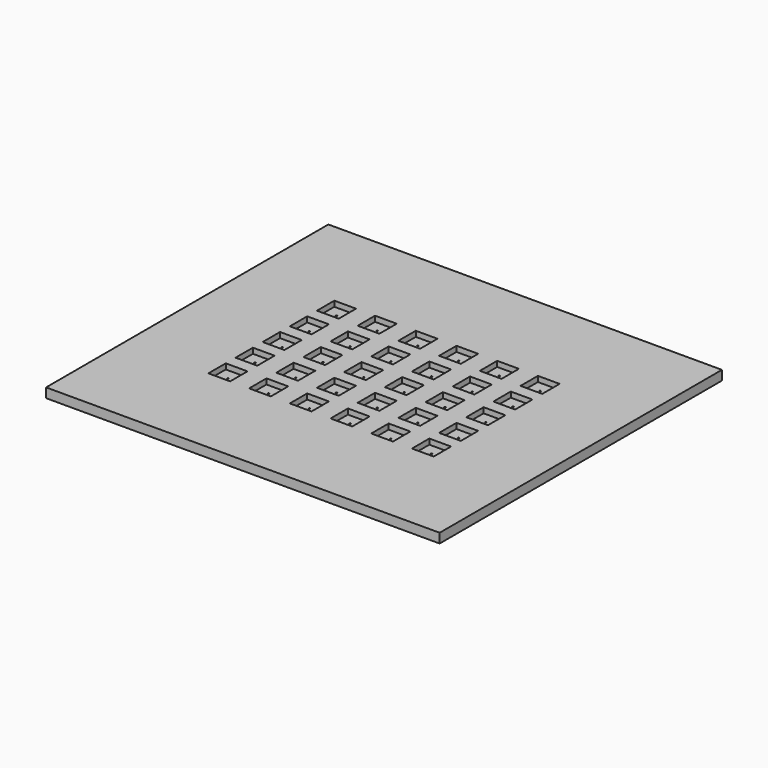
from build123d import *

# Parameters (mm, degrees)
F0_W     = 29
F0_H     = 26
F1_DEPTH = 0.7
F3_W     = 1.6
F3_H     = 1.6
F4_DEPTH = 0.4
F6_D     = 0.1
F8_D     = 0.1
F10_D    = 0.1
F12_D    = 0.1
F14_D    = 0.1
F16_D    = 0.1
F18_D    = 0.1
F20_D    = 0.1
F22_D    = 0.1
F24_D    = 0.1
F26_D    = 0.1
F28_D    = 0.1
F30_D    = 0.1
F32_D    = 0.1
F34_D    = 0.1
F36_D    = 0.1
F38_D    = 0.1
F40_D    = 0.1
F42_D    = 0.1
F44_D    = 0.1
F46_D    = 0.1
F48_D    = 0.1
F50_D    = 0.1
F52_D    = 0.1
F54_D    = 0.1
F56_D    = 0.1
F58_D    = 0.1
F60_D    = 0.1
F62_D    = 0.1
F64_D    = 0.1


# Not quite as in the source:
# - a feature names something its author has since deleted; it is built from what else it names


with BuildPart() as f1:
    # F0 (on Top) → F1 (new body)
    with BuildSketch(Plane.XY):
        Rectangle(F0_W, F0_H)
    extrude(amount=-F1_DEPTH)

    # F3 (on face) → F4 (cut)
    with BuildSketch(Plane.XY):
        with Locations((-7.5, 5)):
            Rectangle(F3_W, F3_H)
        with Locations((-4.5, 5)):
            Rectangle(F3_W, F3_H)
        with Locations((-1.5, 5)):
            Rectangle(F3_W, F3_H)
        with Locations((1.5, 5)):
            Rectangle(F3_W, F3_H)
        with Locations((4.5, 5)):
            Rectangle(F3_W, F3_H)
        with Locations((7.5, 5)):
            Rectangle(F3_W, F3_H)
        with Locations((-7.5, 2.5)):
            Rectangle(F3_W, F3_H)
        with Locations((-4.5, 2.5)):
            Rectangle(F3_W, F3_H)
        with Locations((-1.5, 2.5)):
            Rectangle(F3_W, F3_H)
        with Locations((1.5, 2.5)):
            Rectangle(F3_W, F3_H)
        with Locations((4.5, 2.5)):
            Rectangle(F3_W, F3_H)
        with Locations((7.5, 2.5)):
            Rectangle(F3_W, F3_H)
        with Locations((-7.5, 0)):
            Rectangle(F3_W, F3_H)
        with Locations((-4.5, 0)):
            Rectangle(F3_W, F3_H)
        with Locations((-1.5, 0)):
            Rectangle(F3_W, F3_H)
        with Locations((1.5, 0)):
            Rectangle(F3_W, F3_H)
        with Locations((4.5, 0)):
            Rectangle(F3_W, F3_H)
        with Locations((7.5, 0)):
            Rectangle(F3_W, F3_H)
        with Locations((-7.5, -2.5)):
            Rectangle(F3_W, F3_H)
        with Locations((-4.5, -2.5)):
            Rectangle(F3_W, F3_H)
        with Locations((-1.5, -2.5)):
            Rectangle(F3_W, F3_H)
        with Locations((1.5, -2.5)):
            Rectangle(F3_W, F3_H)
        with Locations((4.5, -2.5)):
            Rectangle(F3_W, F3_H)
        with Locations((7.5, -2.5)):
            Rectangle(F3_W, F3_H)
        with Locations((-7.5, -5)):
            Rectangle(F3_W, F3_H)
        with Locations((-4.5, -5)):
            Rectangle(F3_W, F3_H)
        with Locations((-1.5, -5)):
            Rectangle(F3_W, F3_H)
        with Locations((1.5, -5)):
            Rectangle(F3_W, F3_H)
        with Locations((4.5, -5)):
            Rectangle(F3_W, F3_H)
        with Locations((7.5, -5)):
            Rectangle(F3_W, F3_H)
    extrude(amount=-F4_DEPTH, mode=Mode.SUBTRACT)

    # F6 (through all)
    with Locations(Plane.XY.offset(-0.4)):
        with Locations((-7.5, 5)):
            Hole(F6_D / 2)

    # F8 (through all)
    with Locations(Plane.XY.offset(-0.4)):
        with Locations((-4.5, 5)):
            Hole(F8_D / 2)

    # F10 (through all)
    with Locations(Plane.XY.offset(-0.4)):
        with Locations((-1.5, 5)):
            Hole(F10_D / 2)

    # F12 (through all)
    with Locations(Plane.XY.offset(-0.4)):
        with Locations((1.5, 5)):
            Hole(F12_D / 2)

    # F14 (through all)
    with Locations(Plane.XY.offset(-0.4)):
        with Locations((4.5, 5)):
            Hole(F14_D / 2)

    # F16 (through all)
    with Locations(Plane.XY.offset(-0.4)):
        with Locations((7.5, 5)):
            Hole(F16_D / 2)

    # F18 (through all)
    with Locations(Plane.XY.offset(-0.4)):
        with Locations((7.5, 2.5)):
            Hole(F18_D / 2)

    # F20 (through all)
    with Locations(Plane.XY.offset(-0.4)):
        with Locations((4.5, 2.5)):
            Hole(F20_D / 2)

    # F22 (through all)
    with Locations(Plane.XY.offset(-0.4)):
        with Locations((1.5, 2.5)):
            Hole(F22_D / 2)

    # F24 (through all)
    with Locations(Plane.XY.offset(-0.4)):
        with Locations((-1.5, 2.5)):
            Hole(F24_D / 2)

    # F26 (through all)
    with Locations(Plane.XY.offset(-0.4)):
        with Locations((-4.5, 2.5)):
            Hole(F26_D / 2)

    # F28 (through all)
    with Locations(Plane.XY.offset(-0.4)):
        with Locations((-7.5, 2.5)):
            Hole(F28_D / 2)

    # F30 (through all)
    with Locations(Plane.XY.offset(-0.4)):
        with Locations((-7.5, 0)):
            Hole(F30_D / 2)

    # F32 (through all)
    with Locations(Plane.XY.offset(-0.4)):
        with Locations((-4.5, 0)):
            Hole(F32_D / 2)

    # F34 (through all)
    with Locations(Plane.XY.offset(-0.4)):
        with Locations((-1.5, 0)):
            Hole(F34_D / 2)

    # F36 (through all)
    with Locations(Plane.XY.offset(-0.4)):
        with Locations((1.5, 0)):
            Hole(F36_D / 2)

    # F38 (through all)
    with Locations(Plane.XY.offset(-0.4)):
        with Locations((4.5, 0)):
            Hole(F38_D / 2)

    # F40 (through all)
    with Locations(Plane.XY.offset(-0.4)):
        with Locations((7.5, 0)):
            Hole(F40_D / 2)

    # F42 (through all)
    with Locations(Plane.XY.offset(-0.4)):
        with Locations((-7.5, -2.5)):
            Hole(F42_D / 2)

    # F44 (through all)
    with Locations(Plane.XY.offset(-0.4)):
        with Locations((-4.5, -2.5)):
            Hole(F44_D / 2)

    # F46 (through all)
    with Locations(Plane.XY.offset(-0.4)):
        with Locations((-1.5, -2.5)):
            Hole(F46_D / 2)

    # F48 (through all)
    with Locations(Plane.XY.offset(-0.4)):
        with Locations((1.5, -2.5)):
            Hole(F48_D / 2)

    # F50 (through all)
    with Locations(Plane.XY.offset(-0.4)):
        with Locations((4.5, -2.5)):
            Hole(F50_D / 2)

    # F52 (through all)
    with Locations(Plane.XY.offset(-0.4)):
        with Locations((7.5, -2.5)):
            Hole(F52_D / 2)

    # F54 (through all)
    with Locations(Plane.XY.offset(-0.4)):
        with Locations((7.5, -5)):
            Hole(F54_D / 2)

    # F56 (through all)
    with Locations(Plane.XY.offset(-0.4)):
        with Locations((4.5, -5)):
            Hole(F56_D / 2)

    # F58 (through all)
    with Locations(Plane.XY.offset(-0.4)):
        with Locations((1.5, -5)):
            Hole(F58_D / 2)

    # F60 (through all)
    with Locations(Plane.XY.offset(-0.4)):
        with Locations((-1.5, -5)):
            Hole(F60_D / 2)

    # F62 (through all)
    with Locations(Plane.XY.offset(-0.4)):
        with Locations((-4.5, -5)):
            Hole(F62_D / 2)

    # F64 (through all)
    with Locations(Plane.XY.offset(-0.4)):
        with Locations((-7.5, -5)):
            Hole(F64_D / 2)


solid = f1.part
